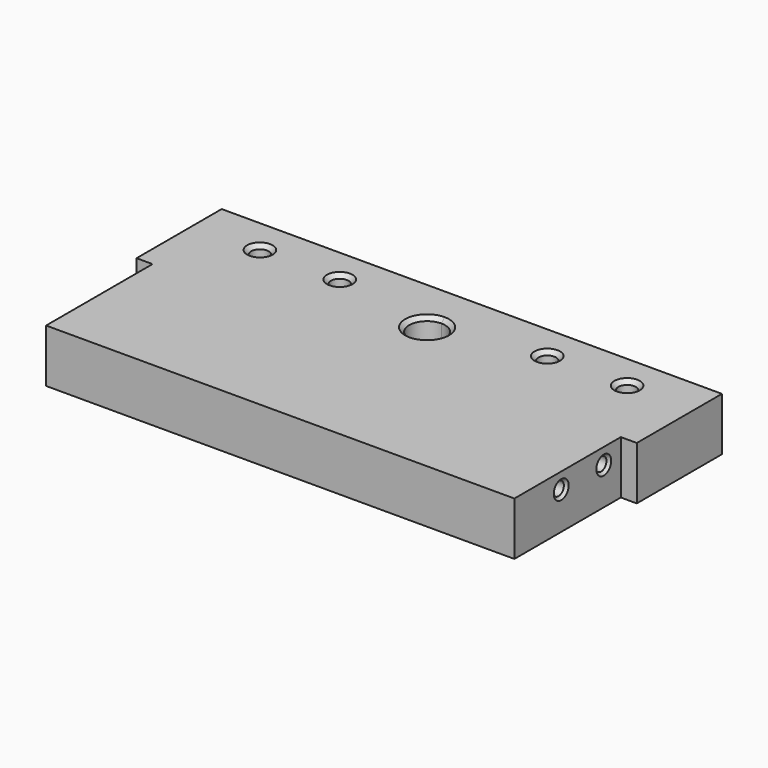
from build123d import *

# Parameters (mm, degrees)
F0_W      = 44
F0_H      = 45
F1_DEPTH  = 10
F2_R      = 1.25
F3_DEPTH  = 88.001
F4_SIZE   = 0.5
F5_W      = 3
F5_H      = 20
F6_DEPTH  = 10
F7_R      = 1.65
F8_DEPTH  = 10.001
F9_SIZE   = 0.75
F10_R     = 1.25
F11_DEPTH = 15
F12_SIZE  = 0.5


with BuildPart() as f1:
    # F0 (on Top) → F1 (new body)
    with BuildSketch(Plane.XY):
        with Locations((-22, 22.5)):
            Rectangle(F0_W, F0_H)
        with Locations((22, 22.5)):
            Rectangle(F0_W, F0_H)
    extrude(amount=F1_DEPTH)

    # F2 (on face) → F3 (cut, through all)
    with BuildSketch(Plane(origin=(-44, 0, 0), x_dir=(0, -1, 0), z_dir=(-1, 0, 0))):
        with Locations((-21, 7)):
            Circle(F2_R)
        with Locations((-11, 7)):
            Circle(F2_R)
    extrude(amount=-F3_DEPTH, mode=Mode.SUBTRACT)

    # F4
    f4_edges = [f1.edges().sort_by_distance(p)[0] for p in [
        (-44, 22.25, 7),
        (-44, 12.25, 7),
        (44, 12.25, 7),
        (44, 22.25, 7),
    ]]
    chamfer(f4_edges, length=F4_SIZE)

    # F5 (on face) → F6 (join, through all)
    with BuildSketch(Plane.XY.offset(10)):
        with Locations((-45.5, 35)):
            Rectangle(F5_W, F5_H)
        with Locations((45.5, 35)):
            Rectangle(F5_W, F5_H)
    extrude(amount=-F6_DEPTH)

    # F7 (on face) → F8 (cut, through all)
    with BuildSketch(Plane.XY.offset(10)):
        with BuildLine():
            Line((0, 31.125), (0, 37.875))
            ThreePointArc((0, 37.875), (-3.375, 34.5), (0, 31.125))
        make_face()
        with BuildLine():
            ThreePointArc((0, 31.125), (2.3864853865, 32.1135146135), (3.375, 34.5))
            ThreePointArc((3.375, 34.5), (2.3864853865, 36.8864853865), (0, 37.875))
            Line((0, 37.875), (0, 31.125))
        make_face()
        with Locations((-34.5, 38.35)):
            Circle(F7_R)
        with BuildLine():
            ThreePointArc((-17.85, 38.35), (-19.5, 40), (-21.15, 38.35))
            ThreePointArc((-21.15, 38.35), (-19.5, 36.7), (-17.85, 38.35))
        make_face()
        with Locations((19.5, 38.35)):
            Circle(F7_R)
        with BuildLine():
            ThreePointArc((36.15, 38.35), (34.5, 40), (32.85, 38.35))
            ThreePointArc((32.85, 38.35), (34.5, 36.7), (36.15, 38.35))
        make_face()
    extrude(amount=-F8_DEPTH, mode=Mode.SUBTRACT)

    # F9
    f9_edges = [f1.edges().sort_by_distance(p)[0] for p in [
        (0, 37.875, 10),
        (0, 37.875, 0),
        (-36.15, 38.35, 10),
        (-17.85, 38.35, 10),
        (17.85, 38.35, 10),
        (36.15, 38.35, 10),
        (36.15, 38.35, 0),
        (17.85, 38.35, 0),
        (-17.85, 38.35, 0),
        (-36.15, 38.35, 0),
    ]]
    chamfer(f9_edges, length=F9_SIZE)

    # F10 (on face) → F11 (cut)
    with BuildSketch(Plane(origin=(0, 45, 0), x_dir=(-1, 0, 0), z_dir=(0, 1, 0))):
        with Locations((-42, 4.9999999996)):
            Circle(F10_R)
        with Locations((42, 4.9999999996)):
            Circle(F10_R)
        with Locations((-27, 4.9999999996)):
            Circle(F10_R)
        with Locations((-12, 4.9999999996)):
            Circle(F10_R)
        with Locations((12, 4.9999999996)):
            Circle(F10_R)
        with Locations((27, 4.9999999996)):
            Circle(F10_R)
    extrude(amount=-F11_DEPTH, mode=Mode.SUBTRACT)

    # F12
    f12_edges = [f1.edges().sort_by_distance(p)[0] for p in [
        (43.25, 45, 5),
        (-40.75, 45, 5),
        (28.25, 45, 5),
        (13.25, 45, 5),
        (-10.75, 45, 5),
        (-25.75, 45, 5),
    ]]
    chamfer(f12_edges, length=F12_SIZE)


solid = f1.part
